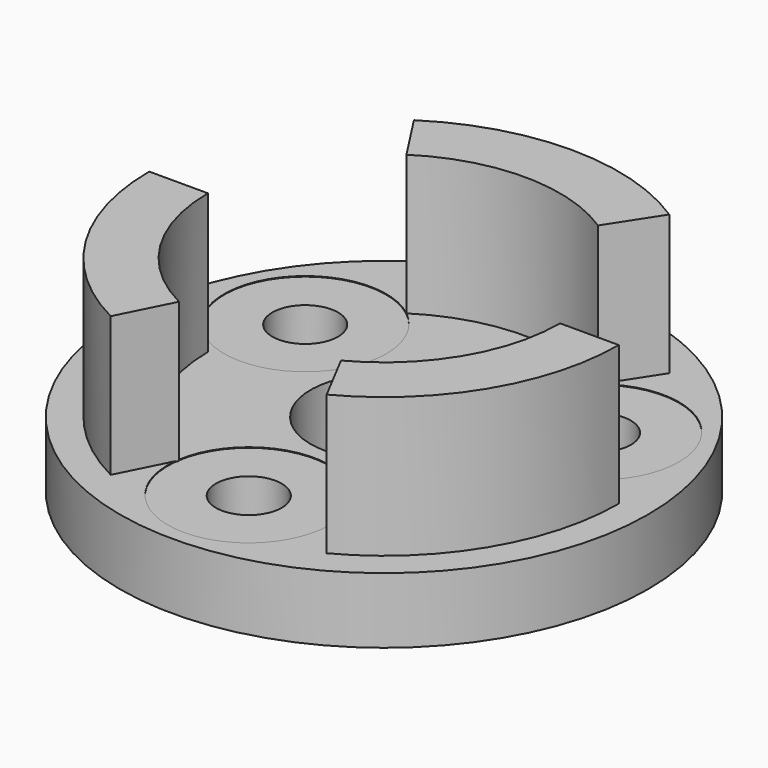
from build123d import *

# Parameters (mm, degrees)
F0_R     = 57.15
F1_DEPTH = 14.224
F3_DEPTH = 30.226
F4_R     = 7.112
F5_DEPTH = 0.127


with BuildPart() as f1:
    # F0 (on Top) → F1 (new body)
    with BuildSketch(Plane.XY):
        Circle(F0_R)
        with BuildLine():
            ThreePointArc((0, -29.464), (5.0289434278, -31.5470565722), (7.112, -36.576))
            ThreePointArc((7.112, -36.576), (-5.0289434278, -41.6049434278), (0, -29.464))
        make_face(mode=Mode.SUBTRACT)
        with BuildLine():
            ThreePointArc((-24.5637451688, 18.288), (-24.8060806923, 16.4472789512), (-25.5165724971, 14.732))
            ThreePointArc((-25.5165724971, 14.732), (-38.5454096454, 20.1287210488), (-24.5637451688, 18.288))
        make_face(mode=Mode.SUBTRACT)
        with BuildLine():
            ThreePointArc((15.875, 0), (11.2253201513, -11.2253201513), (0, -15.875))
            ThreePointArc((0, -15.875), (-13.7481532851, -7.9375), (-13.7481532851, 7.9375))
            ThreePointArc((-13.7481532851, 7.9375), (0, 15.875), (13.7481532851, 7.9375))
            ThreePointArc((13.7481532851, 7.9375), (15.3340724923, 4.108752341), (15.875, 0))
        make_face(mode=Mode.SUBTRACT)
        with BuildLine():
            ThreePointArc((38.7877451688, 18.288), (33.5164662176, 11.4183355234), (25.5165724971, 14.732))
            ThreePointArc((25.5165724971, 14.732), (29.8350241201, 25.1576644766), (38.7877451688, 18.288))
        make_face(mode=Mode.SUBTRACT)
    extrude(amount=F1_DEPTH)

    # F2 (on face) → F3 (join)
    with BuildSketch(Plane.XY.offset(14.224)):
        with BuildLine():
            ThreePointArc((-17.1202854359, -34.0368304428), (-32.4337237695, -19.9915872918), (-38.1, 0))
            Line((-38.1, 0), (-50.8, 0))
            ThreePointArc((-50.8, 0), (-43.244965026, -26.6554497224), (-22.8270472479, -45.3824405904))
            Line((-22.8270472479, -45.3824405904), (-17.1202854359, -34.0368304428))
        make_face()
        with BuildLine():
            ThreePointArc((-20.7239090963, 31.9707615137), (0, 38.1), (20.7239090963, 31.9707615137))
            Line((20.7239090963, 31.9707615137), (27.6318787951, 42.6276820183))
            ThreePointArc((27.6318787951, 42.6276820183), (0, 50.8), (-27.6318787951, 42.6276820183))
            Line((-27.6318787951, 42.6276820183), (-20.7239090963, 31.9707615137))
        make_face()
        with BuildLine():
            ThreePointArc((38.1, 0), (32.6002459501, -19.7188732942), (17.6887682944, -33.7448881496))
            Line((17.6887682944, -33.7448881496), (23.5850243925, -44.9931841994))
            ThreePointArc((23.5850243925, -44.9931841994), (43.4669946002, -26.2918310589), (50.8, 0))
            Line((50.8, 0), (38.1, 0))
        make_face()
    extrude(amount=F3_DEPTH)

    # F4 (on face) → F5 (cut)
    with BuildSketch(Plane.XY.offset(14.224)):
        with BuildLine():
            ThreePointArc((-20.7239090963, 31.9707615137), (-47.4729372454, 10.6979144605), (-14.1497451688, 18.288))
            ThreePointArc((-14.1497451688, 18.288), (-15.8785530923, 25.8780855395), (-20.7239090963, 31.9707615137))
        make_face()
        with Locations((-31.6757451688, 18.288)):
            Circle(F4_R, mode=Mode.SUBTRACT)
        with BuildLine():
            ThreePointArc((49.2017451688, 18.288), (39.2658307083, 34.0851920765), (20.7239090963, 31.9707615137))
            ThreePointArc((20.7239090963, 31.9707615137), (24.0856596293, 2.4908079235), (49.2017451688, 18.288))
        make_face()
        with Locations((31.6757451688, 18.288)):
            Circle(F4_R, mode=Mode.SUBTRACT)
        with BuildLine():
            ThreePointArc((-17.4173370009, -34.6273985025), (-0.9758144603, -54.0748131637), (17.526, -36.576))
            ThreePointArc((17.526, -36.576), (1.3253891442, -19.1001875835), (-17.325537101, -33.9328125))
            ThreePointArc((-17.325537101, -33.9328125), (-17.2229897955, -33.9849764235), (-17.1202854359, -34.0368304428))
            Line((-17.1202854359, -34.0368304428), (-17.4173370009, -34.6273985025))
        make_face()
        with Locations((0, -36.576)):
            Circle(F4_R, mode=Mode.SUBTRACT)
    extrude(amount=-F5_DEPTH, mode=Mode.SUBTRACT)


solid = f1.part
